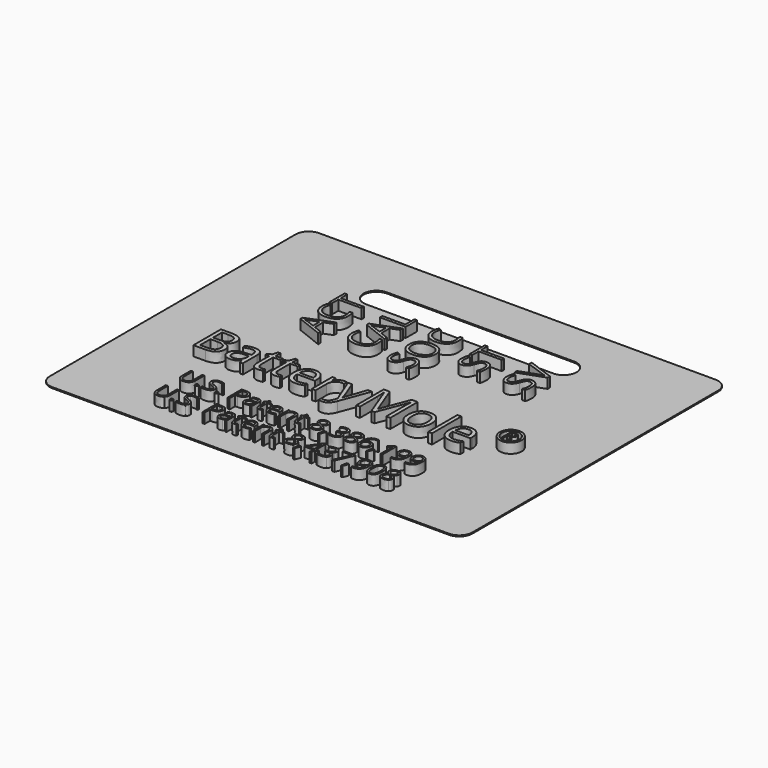
from build123d import *

# Parameters (mm, degrees)
F2_DEPTH       = 0.127
F1_R           = 1.27
F1_R_2         = 1.016
F1_TEXT_SIZE   = 4.1666666667
F1_TEXT_SIZE_2 = 5.5555555556
F1_TEXT_SIZE_3 = 2.0717814957
F1_TEXT_SIZE_4 = 2.8222222222
F3_DEPTH       = 1.27


# Not quite as in the source:
# - Text() gives the source's letters only with a copy of the font that has no kerning and outlines rounded to 1/6400 em; it was checked with that copy


with BuildPart() as f2:
    # F0 (on Top) → F2 (new body)
    with BuildSketch(Plane.XY):
        with BuildLine():
            Line((47.3, 38.5), (1.5, 38.5))
            ThreePointArc((1.5, 38.5), (0.4393398282, 38.0606601718), (0, 37))
            Line((0, 37), (0, 1.5))
            ThreePointArc((0, 1.5), (0.4393398282, 0.4393398282), (1.5, 0))
            Line((1.5, 0), (47.3, 0))
            ThreePointArc((47.3, 0), (48.3606601718, 0.4393398282), (48.8, 1.5))
            Line((48.8, 1.5), (48.8, 37))
            ThreePointArc((48.8, 37), (48.3606601718, 38.0606601718), (47.3, 38.5))
        make_face()
        with BuildLine():
            ThreePointArc((13.5, 30.3), (12, 31.8), (13.5, 33.3))
            Line((13.5, 33.3), (35.1, 33.3))
            ThreePointArc((35.1, 33.3), (36.6, 31.8), (35.1, 30.3))
            Line((35.1, 30.3), (13.5, 30.3))
        make_face(mode=Mode.SUBTRACT)
    extrude(amount=F2_DEPTH)

    # F1 (on Top) → F3 (join)
    with BuildSketch(Plane.XY):
        with Locations((41.1306089235, 16.6292472288)):
            Circle(F1_R)
        with Locations((41.1306089235, 16.6292472288)):
            Circle(F1_R_2, mode=Mode.SUBTRACT)
        with BuildLine():
            add(Edge.make_bspline(
                [(36.4412881944, 3.9645432287), (36.4412881944, 3.4419911453), (36.2765850694, 3.1842428814)],
                knots=[0, 0, 0, 1, 1, 1], degree=2))
            add(Edge.make_bspline(
                [(36.2710729167, 4.7347012148), (36.4412881944, 4.4685744787), (36.4412881944, 3.9645432287)],
                knots=[0, 0, 0, 1, 1, 1], degree=2))
            add(Edge.make_bspline(
                [(35.7727743056, 5.0008279509), (36.1008576389, 5.0008279509), (36.2710729167, 4.7347012148)],
                knots=[0, 0, 0, 1, 1, 1], degree=2))
            add(Edge.make_bspline(
                [(35.2727118056, 4.7457255203), (35.4367534722, 5.0008279509), (35.7727743056, 5.0008279509)],
                knots=[0, 0, 0, 1, 1, 1], degree=2))
            add(Edge.make_bspline(
                [(35.1086701389, 3.9645432287), (35.1086701389, 4.4906230898), (35.2727118056, 4.7457255203)],
                knots=[0, 0, 0, 1, 1, 1], degree=2))
            add(Edge.make_bspline(
                [(35.2782239583, 3.1904164925), (35.1086701389, 3.4543383675), (35.1086701389, 3.9645432287)],
                knots=[0, 0, 0, 1, 1, 1], degree=2))
            add(Edge.make_bspline(
                [(35.7727743056, 2.9264946175), (35.4477777778, 2.9264946175), (35.2782239583, 3.1904164925)],
                knots=[0, 0, 0, 1, 1, 1], degree=2))
            add(Edge.make_bspline(
                [(36.2765850694, 3.1842428814), (36.1118819444, 2.9264946175), (35.7727743056, 2.9264946175)],
                knots=[0, 0, 0, 1, 1, 1], degree=2))
        make_face()
        with BuildLine():
            add(Edge.make_bspline(
                [(35.3401805556, 3.9645432287), (35.3401805556, 3.5248939231), (35.4435885417, 3.324251562)],
                knots=[0, 0, 0, 1, 1, 1], degree=2))
            add(Edge.make_bspline(
                [(35.4435885417, 4.6032914925), (35.3401805556, 4.4041925342), (35.3401805556, 3.9645432287)],
                knots=[0, 0, 0, 1, 1, 1], degree=2))
            add(Edge.make_bspline(
                [(35.7727743056, 4.8023904509), (35.5469965278, 4.8023904509), (35.4435885417, 4.6032914925)],
                knots=[0, 0, 0, 1, 1, 1], degree=2))
            add(Edge.make_bspline(
                [(36.1041649306, 4.6004251731), (36.0016388889, 4.8023904509), (35.7727743056, 4.8023904509)],
                knots=[0, 0, 0, 1, 1, 1], degree=2))
            add(Edge.make_bspline(
                [(36.2066909722, 3.9645432287), (36.2066909722, 4.3984598953), (36.1041649306, 4.6004251731)],
                knots=[0, 0, 0, 1, 1, 1], degree=2))
            add(Edge.make_bspline(
                [(36.1041649306, 3.3268973953), (36.2066909722, 3.5301855898), (36.2066909722, 3.9645432287)],
                knots=[0, 0, 0, 1, 1, 1], degree=2))
            add(Edge.make_bspline(
                [(35.7727743056, 3.1236092009), (36.0016388889, 3.1236092009), (36.1041649306, 3.3268973953)],
                knots=[0, 0, 0, 1, 1, 1], degree=2))
            add(Edge.make_bspline(
                [(35.4435885417, 3.324251562), (35.5469965278, 3.1236092009), (35.7727743056, 3.1236092009)],
                knots=[0, 0, 0, 1, 1, 1], degree=2))
        make_face(mode=Mode.SUBTRACT)
        with BuildLine():
            add(Edge.make_bspline(
                [(37.3862916667, 4.9977411453), (37.6618993056, 4.9977411453), (37.8230746528, 4.8696387148)],
                knots=[0, 0, 0, 1, 1, 1], degree=2))
            add(Edge.make_bspline(
                [(36.9528159722, 4.8676543398), (37.1146527778, 4.9977411453), (37.3862916667, 4.9977411453)],
                knots=[0, 0, 0, 1, 1, 1], degree=2))
            add(Edge.make_bspline(
                [(36.7909791667, 4.5184043398), (36.7909791667, 4.7375675342), (36.9528159722, 4.8676543398)],
                knots=[0, 0, 0, 1, 1, 1], degree=2))
            add(Edge.make_bspline(
                [(36.8736614583, 4.2392689231), (36.7909791667, 4.364064062), (36.7909791667, 4.5184043398)],
                knots=[0, 0, 0, 1, 1, 1], degree=2))
            add(Edge.make_bspline(
                [(37.1464027778, 4.0073175342), (36.95634375, 4.1144737842), (36.8736614583, 4.2392689231)],
                knots=[0, 0, 0, 1, 1, 1], degree=2))
            add(Edge.make_bspline(
                [(36.7248333333, 3.4684494787), (36.7248333333, 3.8141717009), (37.1464027778, 4.0073175342)],
                knots=[0, 0, 0, 1, 1, 1], degree=2))
            add(Edge.make_bspline(
                [(36.8985763889, 3.0678262148), (36.7248333333, 3.209157812), (36.7248333333, 3.4684494787)],
                knots=[0, 0, 0, 1, 1, 1], degree=2))
            add(Edge.make_bspline(
                [(37.3946701389, 2.9264946175), (37.0723194444, 2.9264946175), (36.8985763889, 3.0678262148)],
                knots=[0, 0, 0, 1, 1, 1], degree=2))
            add(Edge.make_bspline(
                [(37.8740069444, 3.076204687), (37.6989409722, 2.9264946175), (37.3946701389, 2.9264946175)],
                knots=[0, 0, 0, 1, 1, 1], degree=2))
            add(Edge.make_bspline(
                [(38.0490729167, 3.4763869787), (38.0490729167, 3.2259147564), (37.8740069444, 3.076204687)],
                knots=[0, 0, 0, 1, 1, 1], degree=2))
            add(Edge.make_bspline(
                [(37.9456649306, 3.7749251731), (38.0490729167, 3.6461612842), (38.0490729167, 3.4763869787)],
                knots=[0, 0, 0, 1, 1, 1], degree=2))
            add(Edge.make_bspline(
                [(37.5970763889, 4.0209876731), (37.8422569444, 3.903689062), (37.9456649306, 3.7749251731)],
                knots=[0, 0, 0, 1, 1, 1], degree=2))
            add(Edge.make_bspline(
                [(37.8920868056, 4.2441196175), (37.7999236111, 4.1215293398), (37.5970763889, 4.0209876731)],
                knots=[0, 0, 0, 1, 1, 1], degree=2))
            add(Edge.make_bspline(
                [(37.98425, 4.5157585064), (37.98425, 4.3667098953), (37.8920868056, 4.2441196175)],
                knots=[0, 0, 0, 1, 1, 1], degree=2))
            add(Edge.make_bspline(
                [(37.8230746528, 4.8696387148), (37.98425, 4.7415362842), (37.98425, 4.5157585064)],
                knots=[0, 0, 0, 1, 1, 1], degree=2))
        make_face()
        with BuildLine():
            add(Edge.make_bspline(
                [(36.9510520833, 3.4627168398), (36.9510520833, 3.2973522564), (37.0659253472, 3.2049685759)],
                knots=[0, 0, 0, 1, 1, 1], degree=2))
            add(Edge.make_bspline(
                [(37.0432152778, 3.7184807287), (36.9510520833, 3.6117654509), (36.9510520833, 3.4627168398)],
                knots=[0, 0, 0, 1, 1, 1], degree=2))
            add(Edge.make_bspline(
                [(37.3408715278, 3.9133904509), (37.1353784722, 3.8251960064), (37.0432152778, 3.7184807287)],
                knots=[0, 0, 0, 1, 1, 1], degree=2))
            add(Edge.make_bspline(
                [(37.7156979167, 3.7114251731), (37.6081006944, 3.8154946175), (37.3408715278, 3.9133904509)],
                knots=[0, 0, 0, 1, 1, 1], degree=2))
            add(Edge.make_bspline(
                [(37.8232951389, 3.4737411453), (37.8232951389, 3.6073557287), (37.7156979167, 3.7114251731)],
                knots=[0, 0, 0, 1, 1, 1], degree=2))
            add(Edge.make_bspline(
                [(37.7088628472, 3.209157812), (37.8232951389, 3.3057307287), (37.8232951389, 3.4737411453)],
                knots=[0, 0, 0, 1, 1, 1], degree=2))
            add(Edge.make_bspline(
                [(37.3889375, 3.1125848953), (37.5944305556, 3.1125848953), (37.7088628472, 3.209157812)],
                knots=[0, 0, 0, 1, 1, 1], degree=2))
            add(Edge.make_bspline(
                [(37.0659253472, 3.2049685759), (37.1807986111, 3.1125848953), (37.3889375, 3.1125848953)],
                knots=[0, 0, 0, 1, 1, 1], degree=2))
        make_face(mode=Mode.SUBTRACT)
        with BuildLine():
            add(Edge.make_bspline(
                [(37.3836458333, 4.8120918398), (37.2112256944, 4.8120918398), (37.1133298611, 4.7294095481)],
                knots=[0, 0, 0, 1, 1, 1], degree=2))
            add(Edge.make_bspline(
                [(37.6585920139, 4.7300710064), (37.5587118056, 4.8120918398), (37.3836458333, 4.8120918398)],
                knots=[0, 0, 0, 1, 1, 1], degree=2))
            add(Edge.make_bspline(
                [(37.7584722222, 4.5087029509), (37.7584722222, 4.6480501731), (37.6585920139, 4.7300710064)],
                knots=[0, 0, 0, 1, 1, 1], degree=2))
            add(Edge.make_bspline(
                [(37.6764513889, 4.2868939231), (37.7584722222, 4.3821439231), (37.7584722222, 4.5087029509)],
                knots=[0, 0, 0, 1, 1, 1], degree=2))
            add(Edge.make_bspline(
                [(37.3973159722, 4.1091821175), (37.5944305556, 4.1916439231), (37.6764513889, 4.2868939231)],
                knots=[0, 0, 0, 1, 1, 1], degree=2))
            add(Edge.make_bspline(
                [(37.0967934028, 4.2910831592), (37.1781527778, 4.2000223953), (37.3973159722, 4.1091821175)],
                knots=[0, 0, 0, 1, 1, 1], degree=2))
            add(Edge.make_bspline(
                [(37.0154340278, 4.5087029509), (37.0154340278, 4.3821439231), (37.0967934028, 4.2910831592)],
                knots=[0, 0, 0, 1, 1, 1], degree=2))
            add(Edge.make_bspline(
                [(37.1133298611, 4.7294095481), (37.0154340278, 4.6467272564), (37.0154340278, 4.5087029509)],
                knots=[0, 0, 0, 1, 1, 1], degree=2))
        make_face(mode=Mode.SUBTRACT)
        with BuildLine():
            add(Edge.make_bspline(
                [(26.3214166667, 4.9977411453), (26.5970243056, 4.9977411453), (26.7581996528, 4.8696387148)],
                knots=[0, 0, 0, 1, 1, 1], degree=2))
            add(Edge.make_bspline(
                [(25.8879409722, 4.8676543398), (26.0497777778, 4.9977411453), (26.3214166667, 4.9977411453)],
                knots=[0, 0, 0, 1, 1, 1], degree=2))
            add(Edge.make_bspline(
                [(25.7261041667, 4.5184043398), (25.7261041667, 4.7375675342), (25.8879409722, 4.8676543398)],
                knots=[0, 0, 0, 1, 1, 1], degree=2))
            add(Edge.make_bspline(
                [(25.8087864583, 4.2392689231), (25.7261041667, 4.364064062), (25.7261041667, 4.5184043398)],
                knots=[0, 0, 0, 1, 1, 1], degree=2))
            add(Edge.make_bspline(
                [(26.0815277778, 4.0073175342), (25.89146875, 4.1144737842), (25.8087864583, 4.2392689231)],
                knots=[0, 0, 0, 1, 1, 1], degree=2))
            add(Edge.make_bspline(
                [(25.6599583333, 3.4684494787), (25.6599583333, 3.8141717009), (26.0815277778, 4.0073175342)],
                knots=[0, 0, 0, 1, 1, 1], degree=2))
            add(Edge.make_bspline(
                [(25.8337013889, 3.0678262148), (25.6599583333, 3.209157812), (25.6599583333, 3.4684494787)],
                knots=[0, 0, 0, 1, 1, 1], degree=2))
            add(Edge.make_bspline(
                [(26.3297951389, 2.9264946175), (26.0074444444, 2.9264946175), (25.8337013889, 3.0678262148)],
                knots=[0, 0, 0, 1, 1, 1], degree=2))
            add(Edge.make_bspline(
                [(26.8091319444, 3.076204687), (26.6340659722, 2.9264946175), (26.3297951389, 2.9264946175)],
                knots=[0, 0, 0, 1, 1, 1], degree=2))
            add(Edge.make_bspline(
                [(26.9841979167, 3.4763869787), (26.9841979167, 3.2259147564), (26.8091319444, 3.076204687)],
                knots=[0, 0, 0, 1, 1, 1], degree=2))
            add(Edge.make_bspline(
                [(26.8807899306, 3.7749251731), (26.9841979167, 3.6461612842), (26.9841979167, 3.4763869787)],
                knots=[0, 0, 0, 1, 1, 1], degree=2))
            add(Edge.make_bspline(
                [(26.5322013889, 4.0209876731), (26.7773819444, 3.903689062), (26.8807899306, 3.7749251731)],
                knots=[0, 0, 0, 1, 1, 1], degree=2))
            add(Edge.make_bspline(
                [(26.8272118056, 4.2441196175), (26.7350486111, 4.1215293398), (26.5322013889, 4.0209876731)],
                knots=[0, 0, 0, 1, 1, 1], degree=2))
            add(Edge.make_bspline(
                [(26.919375, 4.5157585064), (26.919375, 4.3667098953), (26.8272118056, 4.2441196175)],
                knots=[0, 0, 0, 1, 1, 1], degree=2))
            add(Edge.make_bspline(
                [(26.7581996528, 4.8696387148), (26.919375, 4.7415362842), (26.919375, 4.5157585064)],
                knots=[0, 0, 0, 1, 1, 1], degree=2))
        make_face()
        with BuildLine():
            add(Edge.make_bspline(
                [(25.8861770833, 3.4627168398), (25.8861770833, 3.2973522564), (26.0010503472, 3.2049685759)],
                knots=[0, 0, 0, 1, 1, 1], degree=2))
            add(Edge.make_bspline(
                [(25.9783402778, 3.7184807287), (25.8861770833, 3.6117654509), (25.8861770833, 3.4627168398)],
                knots=[0, 0, 0, 1, 1, 1], degree=2))
            add(Edge.make_bspline(
                [(26.2759965278, 3.9133904509), (26.0705034722, 3.8251960064), (25.9783402778, 3.7184807287)],
                knots=[0, 0, 0, 1, 1, 1], degree=2))
            add(Edge.make_bspline(
                [(26.6508229167, 3.7114251731), (26.5432256944, 3.8154946175), (26.2759965278, 3.9133904509)],
                knots=[0, 0, 0, 1, 1, 1], degree=2))
            add(Edge.make_bspline(
                [(26.7584201389, 3.4737411453), (26.7584201389, 3.6073557287), (26.6508229167, 3.7114251731)],
                knots=[0, 0, 0, 1, 1, 1], degree=2))
            add(Edge.make_bspline(
                [(26.6439878472, 3.209157812), (26.7584201389, 3.3057307287), (26.7584201389, 3.4737411453)],
                knots=[0, 0, 0, 1, 1, 1], degree=2))
            add(Edge.make_bspline(
                [(26.3240625, 3.1125848953), (26.5295555556, 3.1125848953), (26.6439878472, 3.209157812)],
                knots=[0, 0, 0, 1, 1, 1], degree=2))
            add(Edge.make_bspline(
                [(26.0010503472, 3.2049685759), (26.1159236111, 3.1125848953), (26.3240625, 3.1125848953)],
                knots=[0, 0, 0, 1, 1, 1], degree=2))
        make_face(mode=Mode.SUBTRACT)
        with BuildLine():
            add(Edge.make_bspline(
                [(26.3187708333, 4.8120918398), (26.1463506944, 4.8120918398), (26.0484548611, 4.7294095481)],
                knots=[0, 0, 0, 1, 1, 1], degree=2))
            add(Edge.make_bspline(
                [(26.5937170139, 4.7300710064), (26.4938368056, 4.8120918398), (26.3187708333, 4.8120918398)],
                knots=[0, 0, 0, 1, 1, 1], degree=2))
            add(Edge.make_bspline(
                [(26.6935972222, 4.5087029509), (26.6935972222, 4.6480501731), (26.5937170139, 4.7300710064)],
                knots=[0, 0, 0, 1, 1, 1], degree=2))
            add(Edge.make_bspline(
                [(26.6115763889, 4.2868939231), (26.6935972222, 4.3821439231), (26.6935972222, 4.5087029509)],
                knots=[0, 0, 0, 1, 1, 1], degree=2))
            add(Edge.make_bspline(
                [(26.3324409722, 4.1091821175), (26.5295555556, 4.1916439231), (26.6115763889, 4.2868939231)],
                knots=[0, 0, 0, 1, 1, 1], degree=2))
            add(Edge.make_bspline(
                [(26.0319184028, 4.2910831592), (26.1132777778, 4.2000223953), (26.3324409722, 4.1091821175)],
                knots=[0, 0, 0, 1, 1, 1], degree=2))
            add(Edge.make_bspline(
                [(25.9505590278, 4.5087029509), (25.9505590278, 4.3821439231), (26.0319184028, 4.2910831592)],
                knots=[0, 0, 0, 1, 1, 1], degree=2))
            add(Edge.make_bspline(
                [(26.0484548611, 4.7294095481), (25.9505590278, 4.6467272564), (25.9505590278, 4.5087029509)],
                knots=[0, 0, 0, 1, 1, 1], degree=2))
        make_face(mode=Mode.SUBTRACT)
        with Locations(Location((36.6, 24.262890625), (0, 0, 90))):
            Text('SV', F1_TEXT_SIZE, font='Open Sans', text_align=(TextAlign.LEFT, TextAlign.BOTTOM))
        with Locations(Location((25.8, 20.993359375), (0, 0, 90))):
            Text('SOC', F1_TEXT_SIZE, font='Open Sans', text_align=(TextAlign.LEFT, TextAlign.BOTTOM))
        with Locations((7.1502256944, 12.6292472288)):
            Text('BatteryMole', F1_TEXT_SIZE_2, font='Open Sans', text_align=(TextAlign.LEFT, TextAlign.BOTTOM))
        with BuildLine():
            add(Edge.make_bspline(
                [(34.8167465278, 4.1091821175), (34.8167465278, 2.9264946175), (33.9017291667, 2.9264946175)],
                knots=[0, 0, 0, 1, 1, 1], degree=2))
            add(Edge.make_bspline(
                [(34.7340642361, 4.5852116314), (34.8167465278, 4.3834668398), (34.8167465278, 4.1091821175)],
                knots=[0, 0, 0, 1, 1, 1], degree=2))
            add(Edge.make_bspline(
                [(34.497703125, 4.8923487842), (34.6513819444, 4.7869564231), (34.7340642361, 4.5852116314)],
                knots=[0, 0, 0, 1, 1, 1], degree=2))
            add(Edge.make_bspline(
                [(34.13853125, 4.9977411453), (34.3440243056, 4.9977411453), (34.497703125, 4.8923487842)],
                knots=[0, 0, 0, 1, 1, 1], degree=2))
            add(Edge.make_bspline(
                [(33.676171875, 4.8158401037), (33.8518993056, 4.9977411453), (34.13853125, 4.9977411453)],
                knots=[0, 0, 0, 1, 1, 1], degree=2))
            add(Edge.make_bspline(
                [(33.5004444444, 4.3199668398), (33.5004444444, 4.633939062), (33.676171875, 4.8158401037)],
                knots=[0, 0, 0, 1, 1, 1], degree=2))
            add(Edge.make_bspline(
                [(33.6576510417, 3.8734824648), (33.5004444444, 4.0333348953), (33.5004444444, 4.3199668398)],
                knots=[0, 0, 0, 1, 1, 1], degree=2))
            add(Edge.make_bspline(
                [(34.0820868056, 3.7136300342), (33.8148576389, 3.7136300342), (33.6576510417, 3.8734824648)],
                knots=[0, 0, 0, 1, 1, 1], degree=2))
            add(Edge.make_bspline(
                [(34.3645295139, 3.7736022564), (34.2390729167, 3.7136300342), (34.0820868056, 3.7136300342)],
                knots=[0, 0, 0, 1, 1, 1], degree=2))
            add(Edge.make_bspline(
                [(34.5658333333, 3.9477862842), (34.4899861111, 3.8335744787), (34.3645295139, 3.7736022564)],
                knots=[0, 0, 0, 1, 1, 1], degree=2))
            Line((34.5658333333, 3.9477862842), (34.5821493056, 3.9477862842))
            add(Edge.make_bspline(
                [(34.3982638889, 3.320282812), (34.56715625, 3.5248939231), (34.5821493056, 3.9477862842)],
                knots=[0, 0, 0, 1, 1, 1], degree=2))
            add(Edge.make_bspline(
                [(33.8986423611, 3.1156717009), (34.2293715278, 3.1156717009), (34.3982638889, 3.320282812)],
                knots=[0, 0, 0, 1, 1, 1], degree=2))
            add(Edge.make_bspline(
                [(33.6481701389, 3.1513904509), (33.7584131944, 3.1156717009), (33.8986423611, 3.1156717009)],
                knots=[0, 0, 0, 1, 1, 1], degree=2))
            Line((33.6481701389, 3.1513904509), (33.6481701389, 2.9542758675))
            add(Edge.make_bspline(
                [(33.9017291667, 2.9264946175), (33.74165625, 2.9264946175), (33.6481701389, 2.9542758675)],
                knots=[0, 0, 0, 1, 1, 1], degree=2))
        make_face()
        with BuildLine():
            add(Edge.make_bspline(
                [(34.13853125, 4.8023904509), (33.9414166667, 4.8023904509), (33.8340399306, 4.675610937)],
                knots=[0, 0, 0, 1, 1, 1], degree=2))
            add(Edge.make_bspline(
                [(34.370703125, 4.7320553814), (34.2695, 4.8023904509), (34.13853125, 4.8023904509)],
                knots=[0, 0, 0, 1, 1, 1], degree=2))
            add(Edge.make_bspline(
                [(34.5285711806, 4.5391300342), (34.47190625, 4.661720312), (34.370703125, 4.7320553814)],
                knots=[0, 0, 0, 1, 1, 1], degree=2))
            add(Edge.make_bspline(
                [(34.5852361111, 4.2719008675), (34.5852361111, 4.4165397564), (34.5285711806, 4.5391300342)],
                knots=[0, 0, 0, 1, 1, 1], degree=2))
            add(Edge.make_bspline(
                [(34.5246024306, 4.0871335064), (34.5852361111, 4.1753279509), (34.5852361111, 4.2719008675)],
                knots=[0, 0, 0, 1, 1, 1], degree=2))
            add(Edge.make_bspline(
                [(34.3585763889, 3.9480067703), (34.46396875, 3.998939062), (34.5246024306, 4.0871335064)],
                knots=[0, 0, 0, 1, 1, 1], degree=2))
            add(Edge.make_bspline(
                [(34.1275069444, 3.8970744787), (34.2531840278, 3.8970744787), (34.3585763889, 3.9480067703)],
                knots=[0, 0, 0, 1, 1, 1], degree=2))
            add(Edge.make_bspline(
                [(33.8258819444, 4.0106248259), (33.9251006944, 3.8970744787), (34.1275069444, 3.8970744787)],
                knots=[0, 0, 0, 1, 1, 1], degree=2))
            add(Edge.make_bspline(
                [(33.7266631944, 4.3226126731), (33.7266631944, 4.1241751731), (33.8258819444, 4.0106248259)],
                knots=[0, 0, 0, 1, 1, 1], degree=2))
            add(Edge.make_bspline(
                [(33.8340399306, 4.675610937), (33.7266631944, 4.5488314231), (33.7266631944, 4.3226126731)],
                knots=[0, 0, 0, 1, 1, 1], degree=2))
        make_face(mode=Mode.SUBTRACT)
        with Locations(Location((31.2, 24.4764322917), (0, 0, 90))):
            Text('ST', F1_TEXT_SIZE, font='Open Sans', text_align=(TextAlign.LEFT, TextAlign.BOTTOM))
        with Locations(Location((15, 21.4979166667), (0, 0, 90))):
            Text('ACT', F1_TEXT_SIZE, font='Open Sans', text_align=(TextAlign.LEFT, TextAlign.BOTTOM))
        with BuildLine():
            add(Edge.make_bspline(
                [(17.7612638889, 4.3821439231), (17.7612638889, 4.0761092009), (17.5524635417, 3.9114060759)],
                knots=[0, 0, 0, 1, 1, 1], degree=2))
            add(Edge.make_bspline(
                [(17.0063194444, 4.9690779509), (17.7612638889, 4.9690779509), (17.7612638889, 4.3821439231)],
                knots=[0, 0, 0, 1, 1, 1], degree=2))
            Line((17.0063194444, 4.9690779509), (16.4837673611, 4.9690779509))
            Line((16.4837673611, 4.9690779509), (16.4837673611, 2.9542758675))
            Line((16.4837673611, 2.9542758675), (16.7179236111, 2.9542758675))
            Line((16.7179236111, 2.9542758675), (16.7179236111, 3.7467029509))
            Line((16.7179236111, 3.7467029509), (16.9551666667, 3.7467029509))
            add(Edge.make_bspline(
                [(17.5524635417, 3.9114060759), (17.3436631944, 3.7467029509), (16.9551666667, 3.7467029509)],
                knots=[0, 0, 0, 1, 1, 1], degree=2))
        make_face()
        with BuildLine():
            Line((16.9291493056, 3.9477862842), (16.7179236111, 3.9477862842))
            Line((16.7179236111, 3.9477862842), (16.7179236111, 4.7662307287))
            Line((16.7179236111, 4.7662307287), (16.9798611111, 4.7662307287))
            add(Edge.make_bspline(
                [(17.3877604167, 4.6685553814), (17.2567916667, 4.7662307287), (16.9798611111, 4.7662307287)],
                knots=[0, 0, 0, 1, 1, 1], degree=2))
            add(Edge.make_bspline(
                [(17.5187291667, 4.3711196175), (17.5187291667, 4.5708800342), (17.3877604167, 4.6685553814)],
                knots=[0, 0, 0, 1, 1, 1], degree=2))
            add(Edge.make_bspline(
                [(17.3796024306, 4.0483279509), (17.5187291667, 4.1488696175), (17.5187291667, 4.3711196175)],
                knots=[0, 0, 0, 1, 1, 1], degree=2))
            add(Edge.make_bspline(
                [(16.9291493056, 3.9477862842), (17.2404756944, 3.9477862842), (17.3796024306, 4.0483279509)],
                knots=[0, 0, 0, 1, 1, 1], degree=2))
        make_face(mode=Mode.SUBTRACT)
        with Locations(Location((20.4, 21.6971354167), (0, 0, 90))):
            Text('CAL', F1_TEXT_SIZE, font='Open Sans', text_align=(TextAlign.LEFT, TextAlign.BOTTOM))
        Polygon((29.0801388889, 3.4172967009), (29.3791180556, 3.4172967009), (29.3791180556, 3.6254355898), (29.0801388889, 3.6254355898), (29.0801388889, 4.9801022564), (28.8376041667, 4.9801022564), (27.8811354167, 3.6170571175), (27.8811354167, 3.4172967009), (28.8609756944, 3.4172967009), (28.8609756944, 2.9542758675), (29.0801388889, 2.9542758675), align=None)
        with BuildLine():
            Line((28.8609756944, 4.2952723953), (28.8609756944, 3.6254355898))
            Line((28.8609756944, 3.6254355898), (28.11, 3.6254355898))
            Line((28.11, 3.6254355898), (28.7397083333, 4.5210501731))
            add(Edge.make_bspline(
                [(28.8640625, 4.7402133675), (28.7979166667, 4.6079217009), (28.7397083333, 4.5210501731)],
                knots=[0, 0, 0, 1, 1, 1], degree=2))
            Line((28.8640625, 4.7402133675), (28.8750868056, 4.7402133675))
            add(Edge.make_bspline(
                [(28.8609756944, 4.2952723953), (28.8609756944, 4.4923869787), (28.8750868056, 4.7402133675)],
                knots=[0, 0, 0, 1, 1, 1], degree=2))
        make_face(mode=Mode.SUBTRACT)
        with BuildLine():
            Line((19.0317048611, 3.169470312), (19.077125, 2.9542758675))
            Line((19.077125, 2.9542758675), (19.2468993056, 2.9542758675))
            Line((19.2468993056, 2.9542758675), (19.2468993056, 3.9852689231))
            add(Edge.make_bspline(
                [(19.1165920139, 4.3695762148), (19.2468993056, 4.2498522564), (19.2468993056, 3.9852689231)],
                knots=[0, 0, 0, 1, 1, 1], degree=2))
            add(Edge.make_bspline(
                [(18.7164097222, 4.4893001731), (18.9862847222, 4.4893001731), (19.1165920139, 4.3695762148)],
                knots=[0, 0, 0, 1, 1, 1], degree=2))
            add(Edge.make_bspline(
                [(18.4494010417, 4.4549043398), (18.5823541667, 4.4893001731), (18.7164097222, 4.4893001731)],
                knots=[0, 0, 0, 1, 1, 1], degree=2))
            add(Edge.make_bspline(
                [(18.2048819444, 4.360095312), (18.3164479167, 4.4205085064), (18.4494010417, 4.4549043398)],
                knots=[0, 0, 0, 1, 1, 1], degree=2))
            Line((18.2048819444, 4.360095312), (18.2754375, 4.1850293398))
            add(Edge.make_bspline(
                [(18.7022986111, 4.300564062), (18.5135625, 4.300564062), (18.2754375, 4.1850293398)],
                knots=[0, 0, 0, 1, 1, 1], degree=2))
            add(Edge.make_bspline(
                [(18.9470381944, 4.2158973953), (18.87075, 4.300564062), (18.7022986111, 4.300564062)],
                knots=[0, 0, 0, 1, 1, 1], degree=2))
            add(Edge.make_bspline(
                [(19.0233263889, 3.9535189231), (19.0233263889, 4.1312307287), (18.9470381944, 4.2158973953)],
                knots=[0, 0, 0, 1, 1, 1], degree=2))
            Line((19.0233263889, 3.9535189231), (19.0233263889, 3.8595918398))
            Line((19.0233263889, 3.8595918398), (18.7671215278, 3.8512133675))
            add(Edge.make_bspline(
                [(18.0355486111, 3.371876562), (18.0355486111, 3.8291647564), (18.7671215278, 3.8512133675)],
                knots=[0, 0, 0, 1, 1, 1], degree=2))
            add(Edge.make_bspline(
                [(18.1629895833, 3.042470312), (18.0355486111, 3.1584460064), (18.0355486111, 3.371876562)],
                knots=[0, 0, 0, 1, 1, 1], degree=2))
            add(Edge.make_bspline(
                [(18.5148854167, 2.9264946175), (18.2904305556, 2.9264946175), (18.1629895833, 3.042470312)],
                knots=[0, 0, 0, 1, 1, 1], degree=2))
            add(Edge.make_bspline(
                [(18.7955642361, 2.976985937), (18.6833368056, 2.9264946175), (18.5148854167, 2.9264946175)],
                knots=[0, 0, 0, 1, 1, 1], degree=2))
            add(Edge.make_bspline(
                [(19.0206805556, 3.169470312), (18.9077916667, 3.0274772564), (18.7955642361, 2.976985937)],
                knots=[0, 0, 0, 1, 1, 1], degree=2))
            Line((19.0206805556, 3.169470312), (19.0317048611, 3.169470312))
        make_face()
        with BuildLine():
            add(Edge.make_bspline(
                [(18.5603055556, 3.1156717009), (18.7741770833, 3.1156717009), (18.8961059028, 3.2327498259)],
                knots=[0, 0, 0, 1, 1, 1], degree=2))
            add(Edge.make_bspline(
                [(18.3504027778, 3.1802741314), (18.4253680556, 3.1156717009), (18.5603055556, 3.1156717009)],
                knots=[0, 0, 0, 1, 1, 1], degree=2))
            add(Edge.make_bspline(
                [(18.2754375, 3.3692307287), (18.2754375, 3.244876562), (18.3504027778, 3.1802741314)],
                knots=[0, 0, 0, 1, 1, 1], degree=2))
            add(Edge.make_bspline(
                [(18.3958229167, 3.6027255203), (18.2754375, 3.5275397564), (18.2754375, 3.3692307287)],
                knots=[0, 0, 0, 1, 1, 1], degree=2))
            add(Edge.make_bspline(
                [(18.7891701389, 3.6876126731), (18.5162083333, 3.6779112842), (18.3958229167, 3.6027255203)],
                knots=[0, 0, 0, 1, 1, 1], degree=2))
            Line((18.7891701389, 3.6876126731), (19.0180347222, 3.6968730898))
            Line((19.0180347222, 3.6968730898), (19.0180347222, 3.5606126731))
            add(Edge.make_bspline(
                [(18.8961059028, 3.2327498259), (19.0180347222, 3.3498279509), (19.0180347222, 3.5606126731)],
                knots=[0, 0, 0, 1, 1, 1], degree=2))
        make_face(mode=Mode.SUBTRACT)
        with BuildLine():
            add(Edge.make_bspline(
                [(21.3521006944, 2.9264946175), (21.0174027778, 2.9264946175), (20.8235954861, 3.1306647564)],
                knots=[0, 0, 0, 1, 1, 1], degree=2))
            add(Edge.make_bspline(
                [(21.61315625, 2.9494251731), (21.5051180556, 2.9264946175), (21.3521006944, 2.9264946175)],
                knots=[0, 0, 0, 1, 1, 1], degree=2))
            add(Edge.make_bspline(
                [(21.8424618056, 3.0243904509), (21.7211944444, 2.9723557287), (21.61315625, 2.9494251731)],
                knots=[0, 0, 0, 1, 1, 1], degree=2))
            Line((21.8424618056, 3.0243904509), (21.8424618056, 3.2285605898))
            add(Edge.make_bspline(
                [(21.3604791667, 3.1266960064), (21.6043368056, 3.1266960064), (21.8424618056, 3.2285605898)],
                knots=[0, 0, 0, 1, 1, 1], degree=2))
            add(Edge.make_bspline(
                [(21.0015277778, 3.2644998259), (21.12896875, 3.1266960064), (21.3604791667, 3.1266960064)],
                knots=[0, 0, 0, 1, 1, 1], degree=2))
            add(Edge.make_bspline(
                [(20.86703125, 3.6682098953), (20.8740868056, 3.4023036453), (21.0015277778, 3.2644998259)],
                knots=[0, 0, 0, 1, 1, 1], degree=2))
            Line((20.86703125, 3.6682098953), (21.9072847222, 3.6682098953))
            Line((21.9072847222, 3.6682098953), (21.9072847222, 3.8128487842))
            add(Edge.make_bspline(
                [(21.7419201389, 4.3056352425), (21.9072847222, 4.1188835064), (21.9072847222, 3.8128487842)],
                knots=[0, 0, 0, 1, 1, 1], degree=2))
            add(Edge.make_bspline(
                [(21.2930104167, 4.4923869787), (21.5765555556, 4.4923869787), (21.7419201389, 4.3056352425)],
                knots=[0, 0, 0, 1, 1, 1], degree=2))
            add(Edge.make_bspline(
                [(20.8097048611, 4.2774130203), (20.9896215278, 4.4923869787), (21.2930104167, 4.4923869787)],
                knots=[0, 0, 0, 1, 1, 1], degree=2))
            add(Edge.make_bspline(
                [(20.6297881944, 3.6968730898), (20.6297881944, 4.062439062), (20.8097048611, 4.2774130203)],
                knots=[0, 0, 0, 1, 1, 1], degree=2))
            add(Edge.make_bspline(
                [(20.8235954861, 3.1306647564), (20.6297881944, 3.3348348953), (20.6297881944, 3.6968730898)],
                knots=[0, 0, 0, 1, 1, 1], degree=2))
        make_face()
        with BuildLine():
            add(Edge.make_bspline(
                [(21.2899236111, 4.300564062), (21.1082430556, 4.300564062), (20.999984375, 4.1821630203)],
                knots=[0, 0, 0, 1, 1, 1], degree=2))
            add(Edge.make_bspline(
                [(21.5657517361, 4.185470312), (21.4693993056, 4.300564062), (21.2899236111, 4.300564062)],
                knots=[0, 0, 0, 1, 1, 1], degree=2))
            add(Edge.make_bspline(
                [(21.6621041667, 3.8543001731), (21.6621041667, 4.070376562), (21.5657517361, 4.185470312)],
                knots=[0, 0, 0, 1, 1, 1], degree=2))
            Line((21.6621041667, 3.8543001731), (20.8723229167, 3.8543001731))
            add(Edge.make_bspline(
                [(20.999984375, 4.1821630203), (20.8917256944, 4.0637619787), (20.8723229167, 3.8543001731)],
                knots=[0, 0, 0, 1, 1, 1], degree=2))
        make_face(mode=Mode.SUBTRACT)
        with BuildLine():
            Line((12.1662083333, 3.665564062), (12.1662083333, 4.9690779509))
            Line((12.1662083333, 4.9690779509), (11.9320520833, 4.9690779509))
            Line((11.9320520833, 4.9690779509), (11.9320520833, 3.6571855898))
            add(Edge.make_bspline(
                [(11.7942482639, 3.2678071175), (11.9320520833, 3.403626562), (11.9320520833, 3.6571855898)],
                knots=[0, 0, 0, 1, 1, 1], degree=2))
            add(Edge.make_bspline(
                [(11.4015625, 3.1319876731), (11.6564444444, 3.1319876731), (11.7942482639, 3.2678071175)],
                knots=[0, 0, 0, 1, 1, 1], degree=2))
            add(Edge.make_bspline(
                [(10.9965295139, 3.2671456592), (11.1343333333, 3.1319876731), (11.4015625, 3.1319876731)],
                knots=[0, 0, 0, 1, 1, 1], degree=2))
            add(Edge.make_bspline(
                [(10.8587256944, 3.6545397564), (10.8587256944, 3.4023036453), (10.9965295139, 3.2671456592)],
                knots=[0, 0, 0, 1, 1, 1], degree=2))
            Line((10.8587256944, 3.6545397564), (10.8587256944, 4.9690779509))
            Line((10.8587256944, 4.9690779509), (10.6241284722, 4.9690779509))
            Line((10.6241284722, 4.9690779509), (10.6241284722, 3.6708557287))
            add(Edge.make_bspline(
                [(10.8232274306, 3.1251526037), (10.6241284722, 3.3238105898), (10.6241284722, 3.6708557287)],
                knots=[0, 0, 0, 1, 1, 1], degree=2))
            add(Edge.make_bspline(
                [(11.3861284722, 2.9264946175), (11.0223263889, 2.9264946175), (10.8232274306, 3.1251526037)],
                knots=[0, 0, 0, 1, 1, 1], degree=2))
            add(Edge.make_bspline(
                [(11.9580694444, 3.1236092009), (11.7499305556, 2.9264946175), (11.3861284722, 2.9264946175)],
                knots=[0, 0, 0, 1, 1, 1], degree=2))
            add(Edge.make_bspline(
                [(12.1662083333, 3.665564062), (12.1662083333, 3.3207237842), (11.9580694444, 3.1236092009)],
                knots=[0, 0, 0, 1, 1, 1], degree=2))
        make_face()
        with Locations((40.4480951614, 15.8901806324)):
            Text('R', F1_TEXT_SIZE_3, font='Open Sans', text_align=(TextAlign.LEFT, TextAlign.BOTTOM))
        with BuildLine():
            add(Edge.make_bspline(
                [(30.8219791667, 4.495032812), (30.8219791667, 4.3018869787), (30.7137204861, 4.1792967009)],
                knots=[0, 0, 0, 1, 1, 1], degree=2))
            add(Edge.make_bspline(
                [(30.6592604167, 4.8634651037), (30.8219791667, 4.729189062), (30.8219791667, 4.495032812)],
                knots=[0, 0, 0, 1, 1, 1], degree=2))
            add(Edge.make_bspline(
                [(30.2032951389, 4.9977411453), (30.4965416667, 4.9977411453), (30.6592604167, 4.8634651037)],
                knots=[0, 0, 0, 1, 1, 1], degree=2))
            add(Edge.make_bspline(
                [(29.8619826389, 4.9419581592), (30.0238194444, 4.9977411453), (30.2032951389, 4.9977411453)],
                knots=[0, 0, 0, 1, 1, 1], degree=2))
            add(Edge.make_bspline(
                [(29.5762326389, 4.7882793398), (29.7001458333, 4.8861751731), (29.8619826389, 4.9419581592)],
                knots=[0, 0, 0, 1, 1, 1], degree=2))
            Line((29.5762326389, 4.7882793398), (29.6917673611, 4.633939062))
            add(Edge.make_bspline(
                [(29.9592170139, 4.7664512148), (29.8421388889, 4.7305119787), (29.6917673611, 4.633939062)],
                knots=[0, 0, 0, 1, 1, 1], degree=2))
            add(Edge.make_bspline(
                [(30.2085868056, 4.8023904509), (30.0762951389, 4.8023904509), (29.9592170139, 4.7664512148)],
                knots=[0, 0, 0, 1, 1, 1], degree=2))
            add(Edge.make_bspline(
                [(30.4835329861, 4.7181647564), (30.3823298611, 4.8023904509), (30.2085868056, 4.8023904509)],
                knots=[0, 0, 0, 1, 1, 1], degree=2))
            add(Edge.make_bspline(
                [(30.5847361111, 4.4866543398), (30.5847361111, 4.633939062), (30.4835329861, 4.7181647564)],
                knots=[0, 0, 0, 1, 1, 1], degree=2))
            add(Edge.make_bspline(
                [(30.4469322917, 4.1978175342), (30.5847361111, 4.3018869787), (30.5847361111, 4.4866543398)],
                knots=[0, 0, 0, 1, 1, 1], degree=2))
            add(Edge.make_bspline(
                [(30.0736493056, 4.0937480898), (30.3091284722, 4.0937480898), (30.4469322917, 4.1978175342)],
                knots=[0, 0, 0, 1, 1, 1], degree=2))
            Line((30.0736493056, 4.0937480898), (29.8725659722, 4.0937480898))
            Line((29.8725659722, 4.0937480898), (29.8725659722, 3.8970744787))
            Line((29.8725659722, 3.8970744787), (30.0710034722, 3.8970744787))
            add(Edge.make_bspline(
                [(30.6469131944, 3.5301855898), (30.6469131944, 3.8970744787), (30.0710034722, 3.8970744787)],
                knots=[0, 0, 0, 1, 1, 1], degree=2))
            add(Edge.make_bspline(
                [(30.1248020833, 3.1209633675), (30.6469131944, 3.1209633675), (30.6469131944, 3.5301855898)],
                knots=[0, 0, 0, 1, 1, 1], degree=2))
            add(Edge.make_bspline(
                [(29.84434375, 3.1546977425), (29.9925104167, 3.1209633675), (30.1248020833, 3.1209633675)],
                knots=[0, 0, 0, 1, 1, 1], degree=2))
            add(Edge.make_bspline(
                [(29.5652083333, 3.2532550342), (29.6961770833, 3.1884321175), (29.84434375, 3.1546977425)],
                knots=[0, 0, 0, 1, 1, 1], degree=2))
            Line((29.5652083333, 3.2532550342), (29.5652083333, 3.0354147564))
            add(Edge.make_bspline(
                [(29.8233975694, 2.9507480898), (29.6904444444, 2.975001562), (29.5652083333, 3.0354147564)],
                knots=[0, 0, 0, 1, 1, 1], degree=2))
            add(Edge.make_bspline(
                [(30.1164236111, 2.9264946175), (29.9563506944, 2.9264946175), (29.8233975694, 2.9507480898)],
                knots=[0, 0, 0, 1, 1, 1], degree=2))
            add(Edge.make_bspline(
                [(30.6839548611, 3.0817168398), (30.4841944444, 2.9264946175), (30.1164236111, 2.9264946175)],
                knots=[0, 0, 0, 1, 1, 1], degree=2))
            add(Edge.make_bspline(
                [(30.8837152778, 3.5248939231), (30.8837152778, 3.236939062), (30.6839548611, 3.0817168398)],
                knots=[0, 0, 0, 1, 1, 1], degree=2))
            add(Edge.make_bspline(
                [(30.7666371528, 3.850110937), (30.8837152778, 3.7259772564), (30.8837152778, 3.5248939231)],
                knots=[0, 0, 0, 1, 1, 1], degree=2))
            add(Edge.make_bspline(
                [(30.4070243056, 4.0042307287), (30.6495590278, 3.9742446175), (30.7666371528, 3.850110937)],
                knots=[0, 0, 0, 1, 1, 1], degree=2))
            Line((30.4070243056, 4.0042307287), (30.4070243056, 4.0152550342))
            add(Edge.make_bspline(
                [(30.7137204861, 4.1792967009), (30.6054618056, 4.0567064231), (30.4070243056, 4.0152550342)],
                knots=[0, 0, 0, 1, 1, 1], degree=2))
        make_face()
        with BuildLine():
            add(Edge.make_bspline(
                [(14.5871458333, 3.4904980898), (14.5871458333, 3.2245918398), (14.3942204861, 3.0755432287)],
                knots=[0, 0, 0, 1, 1, 1], degree=2))
            add(Edge.make_bspline(
                [(14.4680833333, 3.8265189231), (14.5871458333, 3.6968730898), (14.5871458333, 3.4904980898)],
                knots=[0, 0, 0, 1, 1, 1], degree=2))
            add(Edge.make_bspline(
                [(14.0319618056, 4.0690536453), (14.3490208333, 3.9561647564), (14.4680833333, 3.8265189231)],
                knots=[0, 0, 0, 1, 1, 1], degree=2))
            add(Edge.make_bspline(
                [(13.7515034722, 4.1923053814), (13.8432256944, 4.1365223953), (14.0319618056, 4.0690536453)],
                knots=[0, 0, 0, 1, 1, 1], degree=2))
            add(Edge.make_bspline(
                [(13.6211961806, 4.3151161453), (13.65978125, 4.2480883675), (13.7515034722, 4.1923053814)],
                knots=[0, 0, 0, 1, 1, 1], degree=2))
            add(Edge.make_bspline(
                [(13.5826111111, 4.4866543398), (13.5826111111, 4.3821439231), (13.6211961806, 4.3151161453)],
                knots=[0, 0, 0, 1, 1, 1], degree=2))
            add(Edge.make_bspline(
                [(13.6873420139, 4.7084633675), (13.5826111111, 4.6286473953), (13.5826111111, 4.4866543398)],
                knots=[0, 0, 0, 1, 1, 1], degree=2))
            add(Edge.make_bspline(
                [(13.9781631944, 4.7882793398), (13.7920729167, 4.7882793398), (13.6873420139, 4.7084633675)],
                knots=[0, 0, 0, 1, 1, 1], degree=2))
            add(Edge.make_bspline(
                [(14.4632326389, 4.6837689231), (14.2136423611, 4.7882793398), (13.9781631944, 4.7882793398)],
                knots=[0, 0, 0, 1, 1, 1], degree=2))
            Line((14.4632326389, 4.6837689231), (14.5364340278, 4.8874980898))
            add(Edge.make_bspline(
                [(13.9838958333, 4.9977411453), (14.2841979167, 4.9977411453), (14.5364340278, 4.8874980898)],
                knots=[0, 0, 0, 1, 1, 1], degree=2))
            add(Edge.make_bspline(
                [(13.5206545139, 4.8599373259), (13.6955, 4.9977411453), (13.9838958333, 4.9977411453)],
                knots=[0, 0, 0, 1, 1, 1], degree=2))
            add(Edge.make_bspline(
                [(13.3458090278, 4.4893001731), (13.3458090278, 4.7221335064), (13.5206545139, 4.8599373259)],
                knots=[0, 0, 0, 1, 1, 1], degree=2))
            add(Edge.make_bspline(
                [(13.4664149306, 4.1296873259), (13.3458090278, 4.2674911453), (13.3458090278, 4.4893001731)],
                knots=[0, 0, 0, 1, 1, 1], degree=2))
            add(Edge.make_bspline(
                [(13.8679201389, 3.8913418398), (13.5870208333, 3.9918835064), (13.4664149306, 4.1296873259)],
                knots=[0, 0, 0, 1, 1, 1], degree=2))
            add(Edge.make_bspline(
                [(14.1675607639, 3.7632394092), (14.0690034722, 3.8199043398), (13.8679201389, 3.8913418398)],
                knots=[0, 0, 0, 1, 1, 1], degree=2))
            add(Edge.make_bspline(
                [(14.3082309028, 3.639767187), (14.2661180556, 3.7065744787), (14.1675607639, 3.7632394092)],
                knots=[0, 0, 0, 1, 1, 1], degree=2))
            add(Edge.make_bspline(
                [(14.35034375, 3.4684494787), (14.35034375, 3.5729598953), (14.3082309028, 3.639767187)],
                knots=[0, 0, 0, 1, 1, 1], degree=2))
            add(Edge.make_bspline(
                [(14.2317222222, 3.2208435759), (14.35034375, 3.3096994787), (14.35034375, 3.4684494787)],
                knots=[0, 0, 0, 1, 1, 1], degree=2))
            add(Edge.make_bspline(
                [(13.8789444444, 3.1319876731), (14.1131006944, 3.1319876731), (14.2317222222, 3.2208435759)],
                knots=[0, 0, 0, 1, 1, 1], degree=2))
            add(Edge.make_bspline(
                [(13.5896666667, 3.1624147564), (13.7356284722, 3.1319876731), (13.8789444444, 3.1319876731)],
                knots=[0, 0, 0, 1, 1, 1], degree=2))
            add(Edge.make_bspline(
                [(13.3193506944, 3.244876562), (13.4437048611, 3.1928418398), (13.5896666667, 3.1624147564)],
                knots=[0, 0, 0, 1, 1, 1], degree=2))
            Line((13.3193506944, 3.244876562), (13.3193506944, 3.0190987842))
            add(Edge.make_bspline(
                [(13.8705659722, 2.9264946175), (13.5124965278, 2.9264946175), (13.3193506944, 3.0190987842)],
                knots=[0, 0, 0, 1, 1, 1], degree=2))
            add(Edge.make_bspline(
                [(14.3942204861, 3.0755432287), (14.2012951389, 2.9264946175), (13.8705659722, 2.9264946175)],
                knots=[0, 0, 0, 1, 1, 1], degree=2))
        make_face()
        with BuildLine():
            Line((23.3311840278, 3.931470312), (23.3311840278, 2.9542758675))
            Line((23.3311840278, 2.9542758675), (23.5600486111, 2.9542758675))
            Line((23.5600486111, 2.9542758675), (23.5600486111, 3.939407812))
            add(Edge.make_bspline(
                [(23.4222447917, 4.3607567703), (23.5600486111, 4.229126562), (23.5600486111, 3.939407812)],
                knots=[0, 0, 0, 1, 1, 1], degree=2))
            add(Edge.make_bspline(
                [(23.0114791667, 4.4923869787), (23.2844409722, 4.4923869787), (23.4222447917, 4.3607567703)],
                knots=[0, 0, 0, 1, 1, 1], degree=2))
            add(Edge.make_bspline(
                [(22.7290364583, 4.4308713537), (22.8558159722, 4.4923869787), (23.0114791667, 4.4923869787)],
                knots=[0, 0, 0, 1, 1, 1], degree=2))
            add(Edge.make_bspline(
                [(22.5317013889, 4.2577897564), (22.6022569444, 4.3693557287), (22.7290364583, 4.4308713537)],
                knots=[0, 0, 0, 1, 1, 1], degree=2))
            Line((22.5317013889, 4.2577897564), (22.5206770833, 4.2577897564))
            Line((22.5206770833, 4.2577897564), (22.4836354167, 4.4646057287))
            Line((22.4836354167, 4.4646057287), (22.2975451389, 4.4646057287))
            Line((22.2975451389, 4.4646057287), (22.2975451389, 2.9542758675))
            Line((22.2975451389, 2.9542758675), (22.5264097222, 2.9542758675))
            Line((22.5264097222, 2.9542758675), (22.5264097222, 3.7467029509))
            add(Edge.make_bspline(
                [(22.6366527778, 4.1698157981), (22.5264097222, 4.0417133675), (22.5264097222, 3.7467029509)],
                knots=[0, 0, 0, 1, 1, 1], degree=2))
            add(Edge.make_bspline(
                [(22.9836979167, 4.2979182287), (22.7468958333, 4.2979182287), (22.6366527778, 4.1698157981)],
                knots=[0, 0, 0, 1, 1, 1], degree=2))
            add(Edge.make_bspline(
                [(23.2471788194, 4.2068574648), (23.1631736111, 4.2979182287), (22.9836979167, 4.2979182287)],
                knots=[0, 0, 0, 1, 1, 1], degree=2))
            add(Edge.make_bspline(
                [(23.3311840278, 3.931470312), (23.3311840278, 4.1157967009), (23.2471788194, 4.2068574648)],
                knots=[0, 0, 0, 1, 1, 1], degree=2))
        make_face()
        Polygon((32.2767465278, 4.7582932287), (31.4419861111, 2.9542758675), (31.6955451389, 2.9542758675), (32.51928125, 4.7856335064), (32.51928125, 4.9690779509), (31.1787256944, 4.9690779509), (31.1787256944, 4.7582932287), align=None)
        with BuildLine():
            add(Edge.make_bspline(
                [(24.5173993056, 3.1156717009), (24.5782534722, 3.1156717009), (24.6346979167, 3.1244911453)],
                knots=[0, 0, 0, 1, 1, 1], degree=2))
            add(Edge.make_bspline(
                [(24.3396875, 3.1886526037), (24.4045104167, 3.1156717009), (24.5173993056, 3.1156717009)],
                knots=[0, 0, 0, 1, 1, 1], degree=2))
            add(Edge.make_bspline(
                [(24.2748645833, 3.3978939231), (24.2748645833, 3.2616335064), (24.3396875, 3.1886526037)],
                knots=[0, 0, 0, 1, 1, 1], degree=2))
            Line((24.2748645833, 3.3978939231), (24.2748645833, 4.2868939231))
            Line((24.2748645833, 4.2868939231), (24.7131909722, 4.2868939231))
            Line((24.7131909722, 4.2868939231), (24.7131909722, 4.4646057287))
            Line((24.7131909722, 4.4646057287), (24.2748645833, 4.4646057287))
            Line((24.2748645833, 4.4646057287), (24.2748645833, 4.8147376731))
            Line((24.2748645833, 4.8147376731), (24.1425729167, 4.8147376731))
            Line((24.1425729167, 4.8147376731), (24.0464409722, 4.4923869787))
            Line((24.0464409722, 4.4923869787), (23.8299236111, 4.3971369787))
            Line((23.8299236111, 4.3971369787), (23.8299236111, 4.2868939231))
            Line((23.8299236111, 4.2868939231), (24.0464409722, 4.2868939231))
            Line((24.0464409722, 4.2868939231), (24.0464409722, 3.3881925342))
            add(Edge.make_bspline(
                [(24.4843263889, 2.9264946175), (24.0464409722, 2.9264946175), (24.0464409722, 3.3881925342)],
                knots=[0, 0, 0, 1, 1, 1], degree=2))
            add(Edge.make_bspline(
                [(24.6148541667, 2.9384008675), (24.5425347222, 2.9264946175), (24.4843263889, 2.9264946175)],
                knots=[0, 0, 0, 1, 1, 1], degree=2))
            add(Edge.make_bspline(
                [(24.7242152778, 2.9679460064), (24.6871736111, 2.9503071175), (24.6148541667, 2.9384008675)],
                knots=[0, 0, 0, 1, 1, 1], degree=2))
            Line((24.7242152778, 2.9679460064), (24.7242152778, 3.1430119787))
            add(Edge.make_bspline(
                [(24.6346979167, 3.1244911453), (24.6911423611, 3.1333105898), (24.7242152778, 3.1430119787)],
                knots=[0, 0, 0, 1, 1, 1], degree=2))
        make_face()
        with BuildLine():
            add(Edge.make_bspline(
                [(20.2055729167, 3.1156717009), (20.2664270833, 3.1156717009), (20.3228715278, 3.1244911453)],
                knots=[0, 0, 0, 1, 1, 1], degree=2))
            add(Edge.make_bspline(
                [(20.0278611111, 3.1886526037), (20.0926840278, 3.1156717009), (20.2055729167, 3.1156717009)],
                knots=[0, 0, 0, 1, 1, 1], degree=2))
            add(Edge.make_bspline(
                [(19.9630381944, 3.3978939231), (19.9630381944, 3.2616335064), (20.0278611111, 3.1886526037)],
                knots=[0, 0, 0, 1, 1, 1], degree=2))
            Line((19.9630381944, 3.3978939231), (19.9630381944, 4.2868939231))
            Line((19.9630381944, 4.2868939231), (20.4013645833, 4.2868939231))
            Line((20.4013645833, 4.2868939231), (20.4013645833, 4.4646057287))
            Line((20.4013645833, 4.4646057287), (19.9630381944, 4.4646057287))
            Line((19.9630381944, 4.4646057287), (19.9630381944, 4.8147376731))
            Line((19.9630381944, 4.8147376731), (19.8307465278, 4.8147376731))
            Line((19.8307465278, 4.8147376731), (19.7346145833, 4.4923869787))
            Line((19.7346145833, 4.4923869787), (19.5180972222, 4.3971369787))
            Line((19.5180972222, 4.3971369787), (19.5180972222, 4.2868939231))
            Line((19.5180972222, 4.2868939231), (19.7346145833, 4.2868939231))
            Line((19.7346145833, 4.2868939231), (19.7346145833, 3.3881925342))
            add(Edge.make_bspline(
                [(20.1725, 2.9264946175), (19.7346145833, 2.9264946175), (19.7346145833, 3.3881925342)],
                knots=[0, 0, 0, 1, 1, 1], degree=2))
            add(Edge.make_bspline(
                [(20.3030277778, 2.9384008675), (20.2307083333, 2.9264946175), (20.1725, 2.9264946175)],
                knots=[0, 0, 0, 1, 1, 1], degree=2))
            add(Edge.make_bspline(
                [(20.4123888889, 2.9679460064), (20.3753472222, 2.9503071175), (20.3030277778, 2.9384008675)],
                knots=[0, 0, 0, 1, 1, 1], degree=2))
            Line((20.4123888889, 2.9679460064), (20.4123888889, 3.1430119787))
            add(Edge.make_bspline(
                [(20.3228715278, 3.1244911453), (20.3793159722, 3.1333105898), (20.4123888889, 3.1430119787)],
                knots=[0, 0, 0, 1, 1, 1], degree=2))
        make_face()
        with BuildLine():
            Line((33.1657465278, 3.2506092009), (33.1450208333, 3.2823592009))
            Line((33.1450208333, 3.2823592009), (32.8941076389, 3.2823592009))
            add(Edge.make_bspline(
                [(32.8312690972, 2.9445744787), (32.8760277778, 3.1553592009), (32.8941076389, 3.2823592009)],
                knots=[0, 0, 0, 1, 1, 1], degree=2))
            add(Edge.make_bspline(
                [(32.74946875, 2.5904737842), (32.7865104167, 2.7337897564), (32.8312690972, 2.9445744787)],
                knots=[0, 0, 0, 1, 1, 1], degree=2))
            Line((32.74946875, 2.5904737842), (32.9218888889, 2.5904737842))
            add(Edge.make_bspline(
                [(33.0621180556, 2.9300223953), (32.9946493056, 2.7474598953), (32.9218888889, 2.5904737842)],
                knots=[0, 0, 0, 1, 1, 1], degree=2))
            add(Edge.make_bspline(
                [(33.1657465278, 3.2506092009), (33.1295868056, 3.1125848953), (33.0621180556, 2.9300223953)],
                knots=[0, 0, 0, 1, 1, 1], degree=2))
        make_face()
        with BuildLine():
            Line((27.6333090278, 3.2506092009), (27.6125833333, 3.2823592009))
            Line((27.6125833333, 3.2823592009), (27.3616701389, 3.2823592009))
            add(Edge.make_bspline(
                [(27.2988315972, 2.9445744787), (27.3435902778, 3.1553592009), (27.3616701389, 3.2823592009)],
                knots=[0, 0, 0, 1, 1, 1], degree=2))
            add(Edge.make_bspline(
                [(27.21703125, 2.5904737842), (27.2540729167, 2.7337897564), (27.2988315972, 2.9445744787)],
                knots=[0, 0, 0, 1, 1, 1], degree=2))
            Line((27.21703125, 2.5904737842), (27.3894513889, 2.5904737842))
            add(Edge.make_bspline(
                [(27.5296805556, 2.9300223953), (27.4622118056, 2.7474598953), (27.3894513889, 2.5904737842)],
                knots=[0, 0, 0, 1, 1, 1], degree=2))
            add(Edge.make_bspline(
                [(27.6333090278, 3.2506092009), (27.5971493056, 3.1125848953), (27.5296805556, 2.9300223953)],
                knots=[0, 0, 0, 1, 1, 1], degree=2))
        make_face()
        with Locations((10.3705694444, 6.5815989474)):
            Text('U.S. Patent 8,386,199', F1_TEXT_SIZE_4, font='Open Sans', text_align=(TextAlign.LEFT, TextAlign.BOTTOM))
        with BuildLine():
            add(Edge.make_bspline(
                [(12.631875, 3.1002376731), (12.631875, 3.1928418398), (12.6739878472, 3.2402463537)],
                knots=[0, 0, 0, 1, 1, 1], degree=2))
            add(Edge.make_bspline(
                [(12.6779565972, 2.9575831592), (12.631875, 3.0010189231), (12.631875, 3.1002376731)],
                knots=[0, 0, 0, 1, 1, 1], degree=2))
            add(Edge.make_bspline(
                [(12.79459375, 2.9141473953), (12.7240381944, 2.9141473953), (12.6779565972, 2.9575831592)],
                knots=[0, 0, 0, 1, 1, 1], degree=2))
            add(Edge.make_bspline(
                [(12.9185069444, 2.9624338537), (12.8730868056, 2.9141473953), (12.79459375, 2.9141473953)],
                knots=[0, 0, 0, 1, 1, 1], degree=2))
            add(Edge.make_bspline(
                [(12.9639270833, 3.1002376731), (12.9639270833, 3.010720312), (12.9185069444, 2.9624338537)],
                knots=[0, 0, 0, 1, 1, 1], degree=2))
            add(Edge.make_bspline(
                [(12.9191684028, 3.2402463537), (12.9639270833, 3.1928418398), (12.9639270833, 3.1002376731)],
                knots=[0, 0, 0, 1, 1, 1], degree=2))
            add(Edge.make_bspline(
                [(12.79459375, 3.2876508675), (12.8744097222, 3.2876508675), (12.9191684028, 3.2402463537)],
                knots=[0, 0, 0, 1, 1, 1], degree=2))
            add(Edge.make_bspline(
                [(12.6739878472, 3.2402463537), (12.7161006944, 3.2876508675), (12.79459375, 3.2876508675)],
                knots=[0, 0, 0, 1, 1, 1], degree=2))
        make_face()
    extrude(amount=F3_DEPTH)


solid = f2.part
